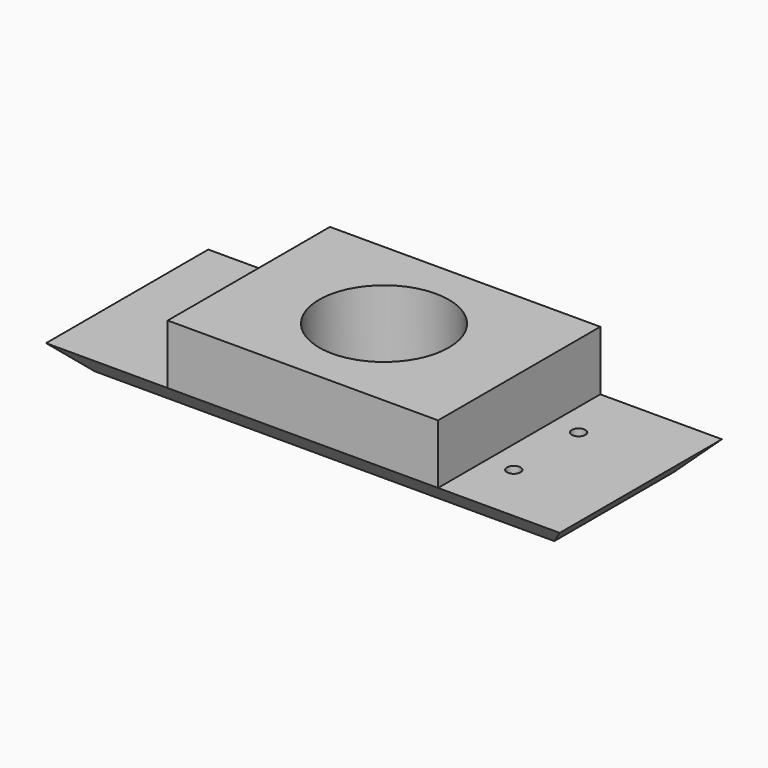
from build123d import *

# Parameters (mm, degrees)
F0_W           = 190
F0_H           = 75
F1_DEPTH       = 10
F2_W           = 100
F2_H           = 75
F3_DEPTH       = 22
F4_R           = 24
F5_DEPTH       = 32.001
F6_SIZE        = 9.99999
F8_D           = 5
F8_CSINK_D     = 9
F8_CSINK_ANGLE = 90


# Not quite as in the source:
# - a fillet or chamfer is up to 0.001 mm smaller than in the source, because OpenCascade refuses the exact size


with BuildPart() as f1:
    # F0 (on Top) → F1 (new body)
    with BuildSketch(Plane.XY):
        Rectangle(F0_W, F0_H)
    extrude(amount=F1_DEPTH)

    # F2 (on face) → F3 (join)
    with BuildSketch(Plane.XY.offset(10)):
        Rectangle(F2_W, F2_H)
    extrude(amount=F3_DEPTH)

    # F4 (on face) → F5 (cut, through all)
    with BuildSketch(Plane.XY.offset(32)):
        Circle(F4_R)
    extrude(amount=-F5_DEPTH, mode=Mode.SUBTRACT)

    # F6 (size 10 in the source; OpenCascade refuses exactly that, so slightly less here)
    f6_edges = [f1.edges().sort_by_distance(p)[0] for p in [
        (95, 0, 0),
        (-95, 0, 0),
        (0, 37.5, 0),
        (0, -37.5, 0),
    ]]
    chamfer(f6_edges, length=F6_SIZE)

    # F8 (through all)
    with Locations(Plane(origin=(0, 0, 0), x_dir=(1, 0, 0), z_dir=(0, 0, -1))):
        with Locations((-60, 15), (-60, -15), (60, 15), (60, -15)):
            CounterSinkHole(F8_D / 2, F8_CSINK_D / 2, counter_sink_angle=F8_CSINK_ANGLE)


solid = f1.part
